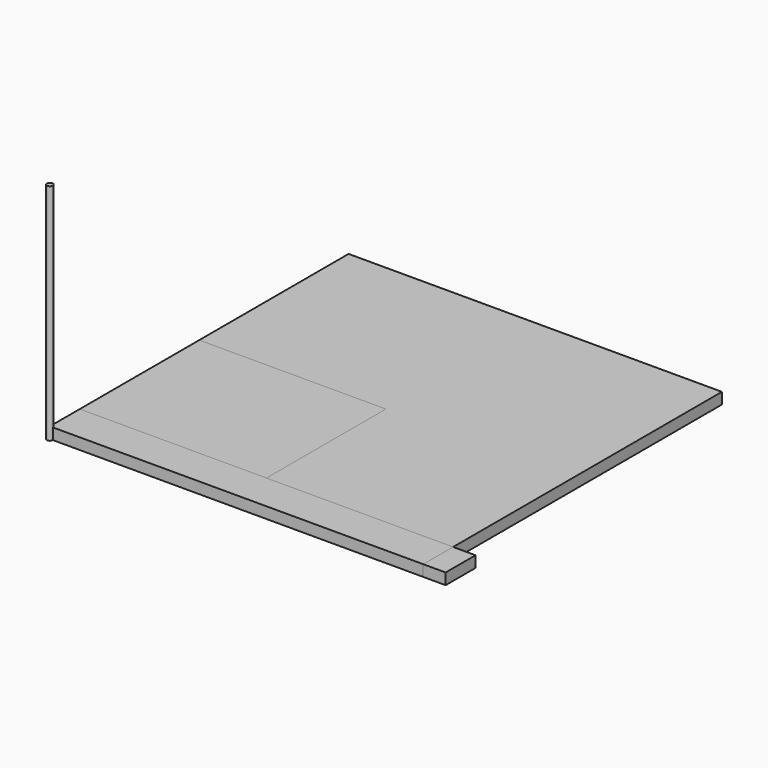
from build123d import *

# Parameters (mm, degrees)
F0_R      = 4
F1_DEPTH  = 300
F2_W      = 500
F2_H      = 42
F3_DEPTH  = 13
F4_W      = 500
F4_H      = 500
F5_DEPTH  = 15
F6_W      = 240
F6_H      = 240
F7_DEPTH  = 1
F8_W      = 50
F8_H      = 250
F9_DEPTH  = 15
F10_W     = 530
F10_H     = 50
F11_DEPTH = 15
F12_W     = 250
F12_H     = 250
F13_DEPTH = 15
F14_W     = 500
F14_H     = 50
F15_DEPTH = 15


# Not quite as in the source:
# - a feature names something its author has since deleted; it is built from what else it names


with BuildPart() as f1:
    # F0 (on Top) → F1 (new body)
    with BuildSketch(Plane.XY):
        Circle(F0_R)
    extrude(amount=F1_DEPTH)


with BuildPart() as f3:
    # F2 (on Top) → F3 (new body)
    with BuildSketch(Plane.XY):
        with Locations((250, 21)):
            Rectangle(F2_W, F2_H)
    extrude(amount=F3_DEPTH)


with BuildPart() as f5:
    # F4 (on Top) → F5 (new body)
    with BuildSketch(Plane.XY):
        with Locations((250, 250)):
            Rectangle(F4_W, F4_H)
    extrude(amount=F5_DEPTH)


with BuildPart() as f7:
    # F6 (on Top) → F7 (new body)
    with BuildSketch(Plane.XY):
        with Locations((120, 120)):
            Rectangle(F6_W, F6_H)
    extrude(amount=F7_DEPTH)


with BuildPart() as f9:
    # F8 (on Top) → F9 (new body)
    with BuildSketch(Plane.XY):
        with Locations((25, 125)):
            Rectangle(F8_W, F8_H)
    extrude(amount=F9_DEPTH)


with BuildPart() as f11:
    # F10 (on Top) → F11 (new body)
    with BuildSketch(Plane.XY):
        with Locations((265, 25)):
            Rectangle(F10_W, F10_H)
    extrude(amount=F11_DEPTH)


with BuildPart() as f13:
    # F12 (on Top) → F13 (new body)
    with BuildSketch(Plane.XY):
        with Locations((125, 125)):
            Rectangle(F12_W, F12_H)
    extrude(amount=F13_DEPTH)


with BuildPart() as f15:
    # F14 (on Top) → F15 (new body)
    with BuildSketch(Plane.XY):
        with Locations((250, 25)):
            Rectangle(F14_W, F14_H)
    extrude(amount=F15_DEPTH)


solid = Compound([f1.part, f3.part, f5.part, f7.part, f9.part, f11.part, f13.part, f15.part])
